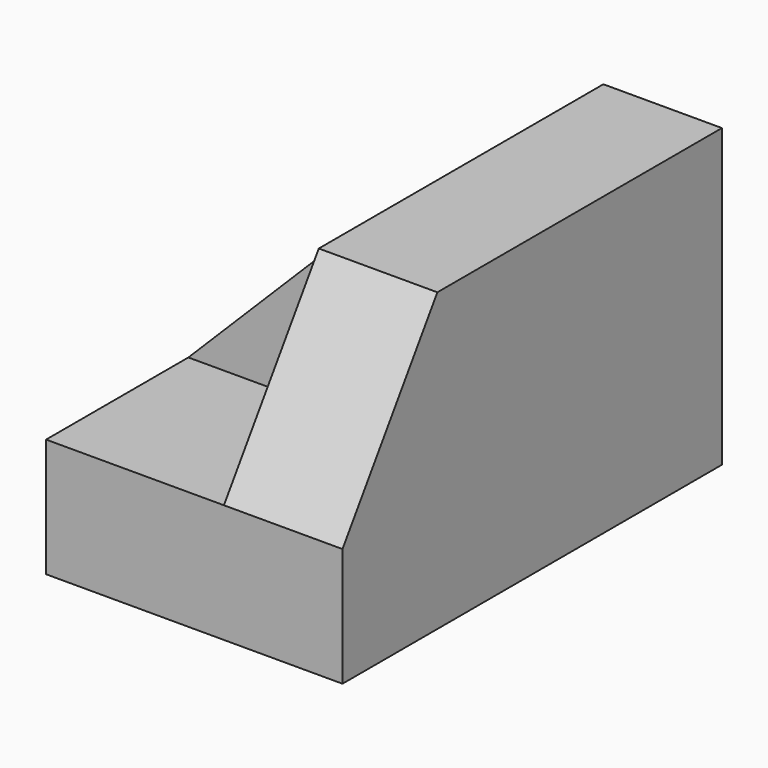
from build123d import *

# Parameters (mm, degrees)
F1_DEPTH = 50.8
F4_DEPTH = 12.7
F2_W     = 19.05
F2_H     = 19.05
F5_DEPTH = 19.05
F7_DEPTH = 12.7
F8_W     = 19.05
F8_H     = 19.05
F9_DEPTH = 19.05


# Not quite as in the source:
# - a feature names something its author has since deleted; it is built from what else it names


with BuildPart() as f1:
    # F0 (on Front) → F1 (new body)
    with BuildSketch(Plane.XZ):
        Polygon((21.3028131574, 38.059670007), (5.7217953451, 38.059670007), (-10.4471868426, 38.059670007), (-10.4471868426, 6.309670007), (21.3028131574, 6.309670007), align=None)
    extrude(amount=F1_DEPTH)

    # F3 (on face) → F4 (cut)
    with BuildSketch(Plane.YZ.offset(21.3028131574)):
        Polygon((-50.8, 38.059670007), (-50.8, 19.009670007), (-38.1, 38.059670007), align=None)
    extrude(amount=-F4_DEPTH, mode=Mode.SUBTRACT)

    # F2 (on face) → F5 (cut)
    with BuildSketch(Plane.XZ.offset(50.8)):
        with Locations((-0.9221868426, 28.534670007)):
            Rectangle(F2_W, F2_H)
    extrude(amount=-F5_DEPTH, mode=Mode.SUBTRACT)

    # F6 (on face) → F7 (cut)
    with BuildSketch(Plane.XZ.offset(31.75)):
        Polygon((-10.4471868426, 19.009670007), (8.6028131574, 38.059670007), (-10.4471868426, 38.059670007), align=None)
    extrude(amount=-F7_DEPTH, mode=Mode.SUBTRACT)

    # F8 (on face) → F9 (cut)
    with BuildSketch(Plane(origin=(0, 0, 0), x_dir=(-1, 0, 0), z_dir=(0, 1, 0))):
        with Locations((0.9221868426, 28.534670007)):
            Rectangle(F8_W, F8_H)
    extrude(amount=-F9_DEPTH, mode=Mode.SUBTRACT)


solid = f1.part
